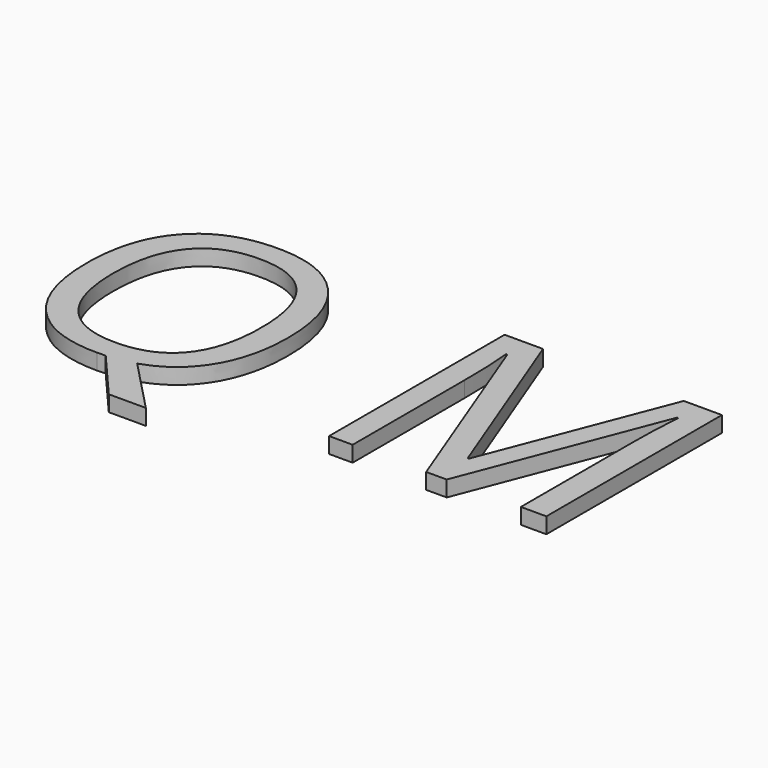
from build123d import *

# Parameters (mm, degrees)
F0_TEXT_SIZE = 123.4722222222
F1_DEPTH     = 6.35


# Not quite as in the source:
# - Text() gives the source's letters only with a copy of the font that has no kerning and outlines rounded to 1/6400 em; it was checked with that copy


with BuildPart() as f1:
    # F0 (on Top) → F1 (new body)
    with BuildSketch(Plane.XY):
        with Locations((-72.5616205581, -59.947431865)):
            Text('Q M', F0_TEXT_SIZE, font='Open Sans', text_align=(TextAlign.LEFT, TextAlign.BOTTOM))
    extrude(amount=F1_DEPTH)


solid = f1.part
